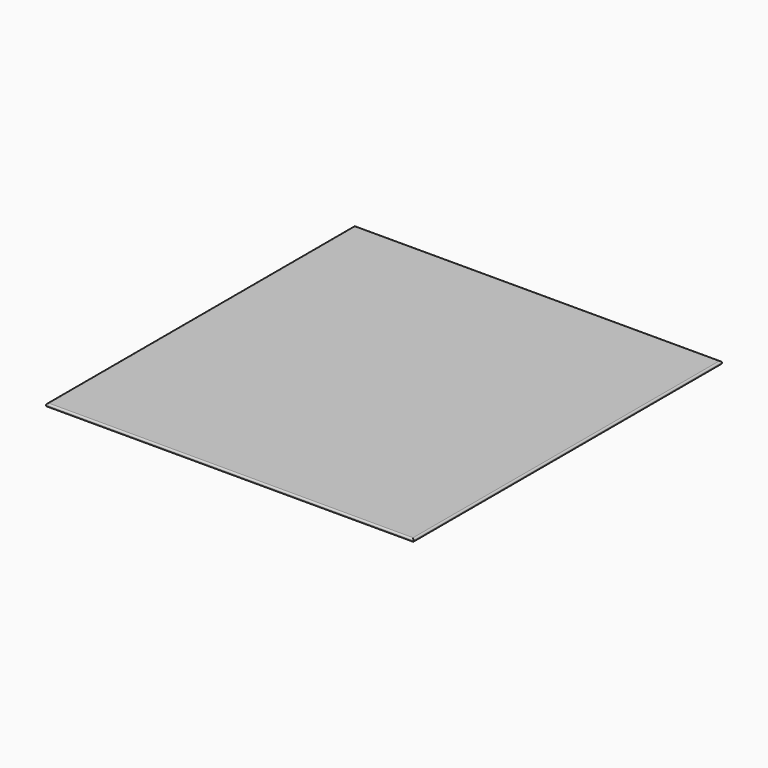
from build123d import *

# Parameters (mm, degrees)
F0_W     = 2032
F0_H     = 2133.6
F1_DEPTH = 17.78
F2_R     = 8.88999


# Not quite as in the source:
# - a fillet or chamfer is up to 0.001 mm smaller than in the source, because OpenCascade refuses the exact size


with BuildPart() as f1:
    # F0 (on Top) → F1 (new body)
    with BuildSketch(Plane.XY):
        Rectangle(F0_W, F0_H)
    extrude(amount=-F1_DEPTH)

    # F2 (radius 8.89 in the source; OpenCascade refuses exactly that, so slightly less here)
    f2_edges = [f1.edges().sort_by_distance(p)[0] for p in [
        (1016, 0, 0),
        (0, 1066.8, 0),
        (-1016, 0, 0),
        (0, -1066.8, 0),
        (0, -1066.8, -17.78),
        (-1016, 0, -17.78),
        (0, 1066.8, -17.78),
        (1016, 0, -17.78),
    ]]
    fillet(f2_edges, radius=F2_R)


solid = f1.part
